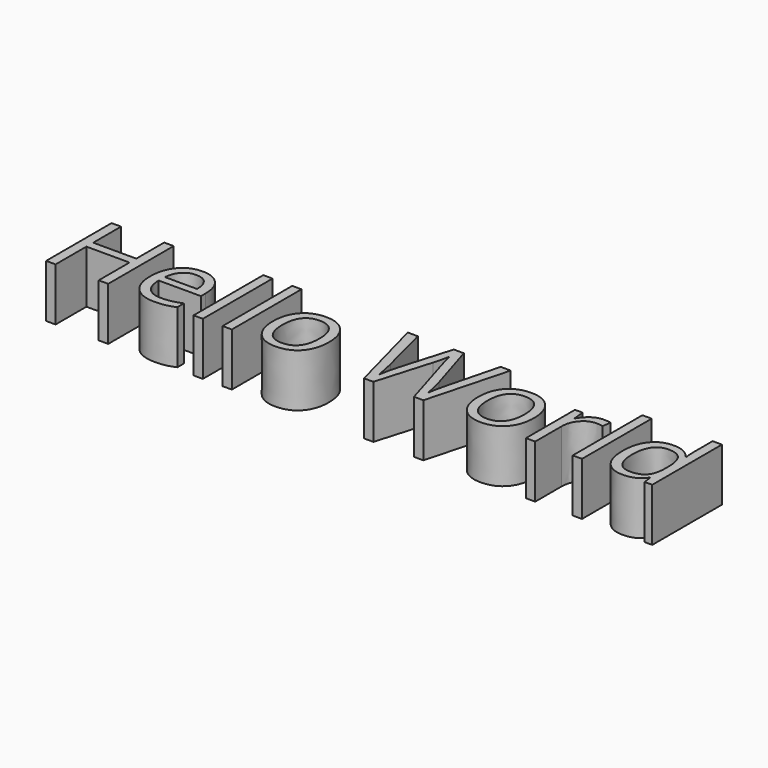
from build123d import *

# Parameters (mm, degrees)
F0_TEXT_SIZE = 55.0042579157
F1_DEPTH     = 25.4


# Not quite as in the source:
# - Text() gives the source's letters only with a copy of the font that has no kerning and outlines rounded to 1/6400 em; it was checked with that copy


with BuildPart() as f1:
    # F0 (on Top) → F1 (new body)
    with BuildSketch(Plane.XY):
        with Locations((0, 0)):
            Text('Hello World', F0_TEXT_SIZE, font='Open Sans', text_align=(TextAlign.LEFT, TextAlign.BOTTOM))
    extrude(amount=F1_DEPTH)


solid = f1.part
